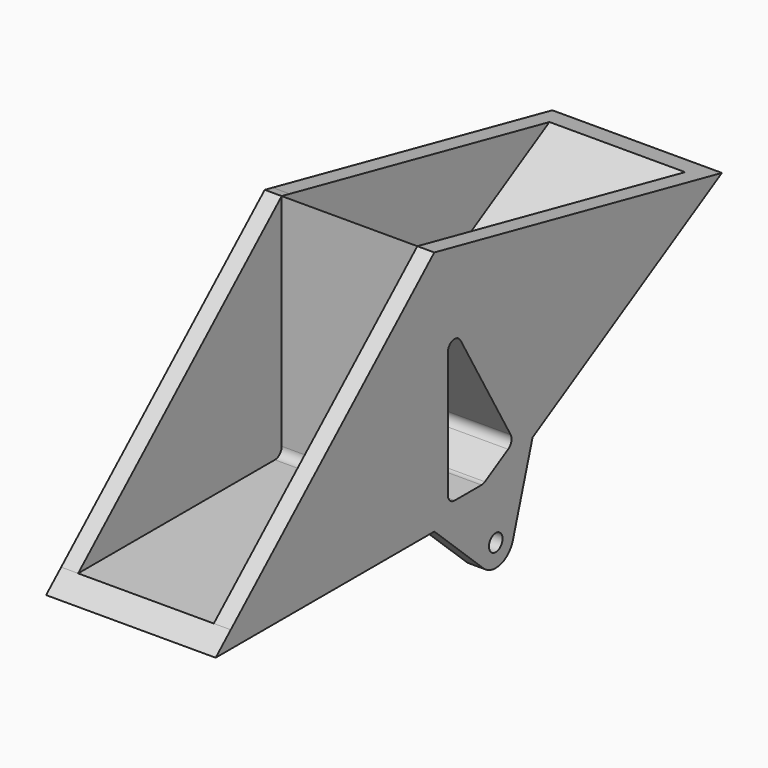
from build123d import *

# Parameters (mm, degrees)
F0_R     = 1.27
F1_DEPTH = 25.4
F2_DEPTH = 2.54
F4_DEPTH = 2.54
F8_DEPTH = 20.32


# Not quite as in the source:
# - a feature names something its author has since deleted; it is built from what else it names


with BuildPart() as f1:
    # F0 (on Right) → F1 (new body)
    with BuildSketch(Plane.YZ):
        with BuildLine():
            Line((-50.8, 0), (-9.8610056184, 0))
            Line((-9.8610056184, 0), (-0.6510920475, -8.592966345))
            ThreePointArc((-0.6510920475, -8.592966345), (2.514052834, -9.3825729095), (4.8603454258, -7.1161811248))
            Line((4.8603454258, -7.1161811248), (8.5398813724, 4.9305028092))
            Line((8.5398813724, 4.9305028092), (43.9940905122, 25.4))
            Line((43.9940905122, 25.4), (40.2770972977, 26.1869323345))
            Line((40.2770972977, 26.1869323345), (8.3697336352, 7.7652073348))
            ThreePointArc((8.3697336352, 7.7652073348), (7.4060334479, 7.6383337982), (6.6348813724, 8.2300595976))
            Line((6.6348813724, 8.2300595976), (-9.8610056184, 36.8017739816))
            Line((-9.8610056184, 36.8017739816), (-9.8610056184, 3.81))
            ThreePointArc((-9.8610056184, 3.81), (-10.2329800063, 2.9119743879), (-11.1310056184, 2.54))
            Line((-11.1310056184, 2.54), (-47.9744556178, 2.54))
            Line((-47.9744556178, 2.54), (-50.8, 0))
        make_face()
        with Locations((1.6435009364, -6.1336289969)):
            Circle(F0_R, mode=Mode.SUBTRACT)
        with BuildLine():
            Line((-1.0208864232, 2.54), (-6.0510056184, 2.54))
            ThreePointArc((-6.0510056184, 2.54), (-6.9490312305, 2.9119743879), (-7.3210056184, 3.81))
            Line((-7.3210056184, 3.81), (-7.3210056184, 22.5826604048))
            ThreePointArc((-7.3210056184, 22.5826604048), (-6.3797058057, 23.8093862042), (-4.9511533556, 23.2176604048))
            Line((-4.9511533556, 23.2176604048), (4.4351768468, 6.9600595976))
            ThreePointArc((4.4351768468, 6.9600595976), (4.5620503834, 5.9963594103), (3.970324584, 5.2252073348))
            Line((3.970324584, 5.2252073348), (-0.3858864232, 2.7101477372))
            ThreePointArc((-0.3858864232, 2.7101477372), (-0.6921862359, 2.5832742006), (-1.0208864232, 2.54))
        make_face(mode=Mode.SUBTRACT)
    extrude(amount=F1_DEPTH)

    # F0 (on Right) → F2 (join)
    with BuildSketch(Plane.YZ):
        with BuildLine():
            Line((-9.8610056184, 36.8017739816), (-47.9744556178, 2.54))
            Line((-47.9744556178, 2.54), (-11.1310056184, 2.54))
            ThreePointArc((-11.1310056184, 2.54), (-10.2329800063, 2.9119743879), (-9.8610056184, 3.81))
            Line((-9.8610056184, 3.81), (-9.8610056184, 36.8017739816))
        make_face()
        with BuildLine():
            Line((-8.3631146249, 36.484652376), (-9.8610056184, 36.8017739816))
            Line((-9.8610056184, 36.8017739816), (6.6348813724, 8.2300595976))
            ThreePointArc((6.6348813724, 8.2300595976), (7.4060334479, 7.6383337982), (8.3697336352, 7.7652073348))
            Line((8.3697336352, 7.7652073348), (40.2770972977, 26.1869323345))
            Line((40.2770972977, 26.1869323345), (-8.3631146249, 36.484652376))
        make_face()
    extrude(amount=F2_DEPTH)

    # F3 (on face) → F4 (join)
    with BuildSketch(Plane.YZ.offset(25.4)):
        with BuildLine():
            Line((-9.8610056184, 3.81), (-9.8610056184, 36.8017739816))
            Line((-9.8610056184, 36.8017739816), (-47.9744556178, 2.54))
            Line((-47.9744556178, 2.54), (-11.1310056184, 2.54))
            ThreePointArc((-11.1310056184, 2.54), (-10.2329800063, 2.9119743879), (-9.8610056184, 3.81))
        make_face()
        with BuildLine():
            Line((40.2770972977, 26.1869323345), (-9.8610056184, 36.8017739816))
            Line((-9.8610056184, 36.8017739816), (6.6348813724, 8.2300595976))
            ThreePointArc((6.6348813724, 8.2300595976), (7.4060334479, 7.6383337982), (8.3697336352, 7.7652073348))
            Line((8.3697336352, 7.7652073348), (40.2770972977, 26.1869323345))
        make_face()
    extrude(amount=-F4_DEPTH)

    # F7 (on offset) → F8 (cut)
    with BuildSketch(Plane.YZ.offset(2.54)):
        with BuildLine():
            Line((8.5398813724, 4.9305028092), (0.2947045256, 0.1701477372))
            ThreePointArc((0.2947045256, 0.1701477372), (-0.0115952871, 0.0432742006), (-0.3402954744, 0))
            Line((-0.3402954744, 0), (-9.8610056184, 0))
            Line((-9.8610056184, 0), (-0.6510920475, -8.592966345))
            ThreePointArc((-0.6510920475, -8.592966345), (2.514052834, -9.3825729095), (4.8603454258, -7.1161811248))
            Line((4.8603454258, -7.1161811248), (8.5398813724, 4.9305028092))
        make_face()
    extrude(amount=F8_DEPTH, mode=Mode.SUBTRACT)


solid = f1.part
